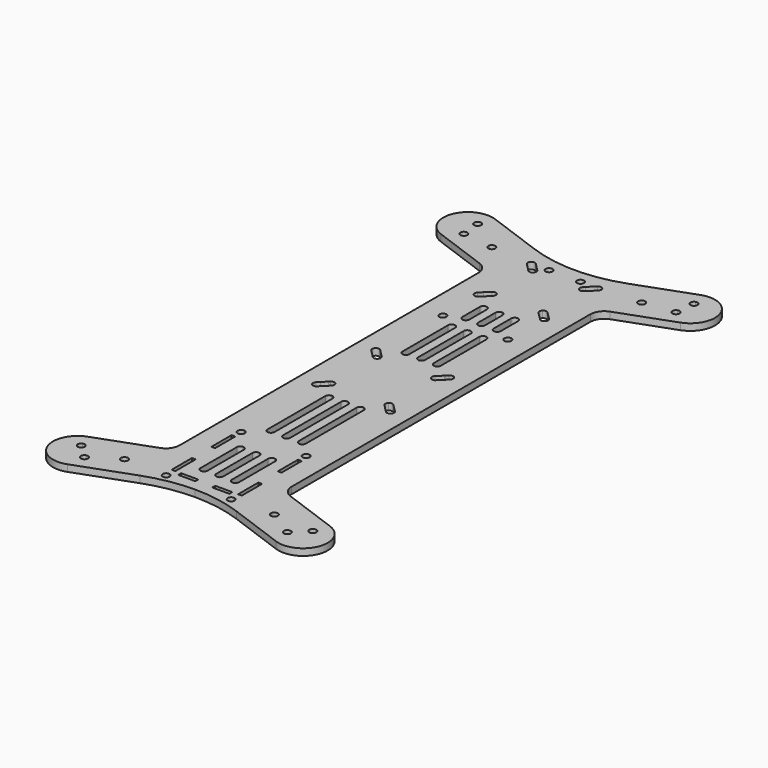
from build123d import *

# Parameters (mm, degrees)
F0_W     = 3.775
F0_H     = 1
F0_W_2   = 0.5
F0_H_2   = 10.85
F0_W_3   = 3.85
F0_H_3   = 25.4769915305
F0_H_4   = 9.7843557596
F0_H_5   = 20.2333889902
F1_DEPTH = 3


# Not quite as in the source:
# - a feature names something its author has since deleted; it is built from what else it names


with BuildPart() as f1:
    # F0 (on Top) → F1 (new body)
    with BuildSketch(Plane.XY):
        with Locations((6.6657602992, -80.0343685785)):
            Rectangle(F0_W, F0_H)
        with BuildLine():
            ThreePointArc((58.190047871, 117.9808986768), (64.7644140361, 132.0798244914), (50.6654338992, 138.6540741594))
            Line((50.6654338992, 138.6540741594), (52.5342574987, 133.5195235187))
            ThreePointArc((52.5342574987, 133.5195235187), (53.9763221117, 133.3296721108), (54.6479392245, 132.039507641))
            ThreePointArc((54.6479392245, 132.039507641), (54.3631036942, 131.1361247537), (53.6116209502, 130.5594917633))
            Line((53.6116209502, 130.5594917633), (54.7696756191, 127.37776271))
            Line((54.7696756191, 127.37776271), (58.190047871, 117.9808986768))
        make_face()
        with BuildLine():
            Line((36.7554780085, 120.8211309856), (29.7782602992, 118.2816314214))
            Line((29.778260321, 118.2816314276), (33.1987034785, 108.8847932036))
            Line((33.1987034785, 108.8847932036), (33.8827906821, 109.1337805834))
            Line((33.8827906821, 109.1337805834), (58.190047871, 117.9808986768))
            Line((58.190047871, 117.9808986768), (54.7696756191, 127.37776271))
            Line((54.7696756191, 127.37776271), (51.1158606394, 126.0478828159))
            Line((51.1158606394, 126.0478828159), (39.715509764, 121.8984944371))
            ThreePointArc((39.715509764, 121.8984944371), (39.7865660973, 121.6333085911), (39.8104938863, 121.3598127113))
            ThreePointArc((39.8104938863, 121.3598127113), (38.5089897661, 119.8087405003), (36.7554780085, 120.8211309856))
        make_face()
        with BuildLine():
            ThreePointArc((53.7365490928, 123.1748774023), (51.2581662055, 121.8847129326), (51.6228673671, 124.6548932801))
            ThreePointArc((51.6228673671, 124.6548932801), (53.06493198, 124.4650418721), (53.7365490928, 123.1748774023))
        make_face(mode=Mode.SUBTRACT)
        Polygon((33.1987034785, 108.8847932036), (29.778260321, 118.2816314276), (29.7782602992, 107.6398536984), align=None)
        with BuildLine():
            Line((14.9782756182, 115.4816467686), (9.7782603038, 110.2816314563))
            Line((9.7782603038, 110.2816314563), (9.7782603038, 100.281631451))
            Line((9.7782603038, 100.281631451), (14.9782756245, 95.0816161323))
            ThreePointArc((14.9782756245, 95.0816161323), (16.0919688055, 95.5429229525), (17.2056619867, 95.0816161328))
            Line((17.2056619867, 95.0816161328), (19.2782602992, 93.0090178203))
            Line((19.2782602992, 93.0090178203), (19.2782602992, 117.554245087))
            Line((19.2782602992, 117.554245087), (17.2056619804, 115.4816467682))
            ThreePointArc((17.2056619804, 115.4816467682), (16.0919687992, 115.0203399485), (14.9782756182, 115.4816467686))
        make_face()
        with BuildLine():
            Line((11.7782603087, 118.2816314214), (4.7782602992, 118.2816314214))
            Line((4.7782602992, 118.2816314214), (4.7782602992, 110.2816314563))
            Line((4.7782602992, 110.2816314563), (9.7782603038, 110.2816314563))
            Line((9.7782603038, 110.2816314563), (14.9782756182, 115.4816467686))
            ThreePointArc((14.9782756182, 115.4816467686), (14.5169687985, 116.5953399498), (14.9782756187, 117.7090331308))
            Line((14.9782756187, 117.7090331308), (15.5508739097, 118.2816314214))
            Line((15.5508739097, 118.2816314214), (11.7782603087, 118.2816314214))
        make_face()
        Polygon((9.7782603038, 110.2816314563), (4.7782602992, 110.2816314563), (4.7782602992, 105.2816314536), align=None)
        Polygon((9.7782603038, 110.2816314563), (4.7782602992, 105.2816314536), (9.7782603038, 100.281631451), align=None)
        Polygon((9.7782603038, 100.281631451), (4.7782602992, 105.2816314536), (4.7782602992, 100.281631451), align=None)
        with BuildLine():
            Line((9.7782603038, 100.281631451), (4.7782602992, 100.281631451))
            Line((4.7782602992, 100.281631451), (4.7782602992, 85.1705366492))
            ThreePointArc((4.7782602992, 85.1705366492), (5.8919534795, 84.7092298296), (6.3532602992, 83.5955366492))
            Line((6.3532602992, 83.5955366492), (10.2032602992, 83.5955366492))
            ThreePointArc((10.2032602992, 83.5955366492), (11.7782602992, 85.1705366492), (13.3532602992, 83.5955366492))
            Line((13.3532602992, 83.5955366492), (19.2782602992, 83.5955366492))
            Line((19.2782602992, 83.5955366492), (19.2782602992, 88.896597805))
            ThreePointArc((19.2782602992, 88.896597805), (18.866196709, 89.053607639), (18.5138095323, 89.3186958657))
            Line((18.5138095323, 89.3186958657), (14.978275625, 92.8542297702))
            ThreePointArc((14.978275625, 92.8542297702), (14.5169688048, 93.9679229512), (14.9782756245, 95.0816161323))
            Line((14.9782756245, 95.0816161323), (9.7782603038, 100.281631451))
        make_face()
        with BuildLine():
            Line((16.6290332129, 32.9517906959), (19.0508739384, 35.3736314215))
            Line((19.0508739384, 35.3736314215), (11.7782602992, 35.3736314215))
            Line((11.7782602992, 35.3736314215), (11.7782602992, 25.8736314215))
            Line((11.7782602992, 25.8736314215), (16.6290332129, 30.7244043352))
            ThreePointArc((16.6290332129, 30.7244043352), (16.1677263933, 31.8380975156), (16.6290332129, 32.9517906959))
        make_face()
        with BuildLine():
            Line((16.6290332129, 7.0228585078), (11.7782602992, 11.8736314215))
            Line((11.7782602992, 11.8736314215), (11.7782602992, 2.3736314215))
            Line((11.7782602992, 2.3736314215), (19.0508739384, 2.3736314215))
            Line((19.0508739384, 2.3736314215), (16.6290332129, 4.795472147))
            ThreePointArc((16.6290332129, 4.795472147), (16.1677263933, 5.9091653274), (16.6290332129, 7.0228585078))
        make_face()
        with BuildLine():
            Line((29.7782602992, -63.3962838112), (29.7782602992, 18.8736314215))
            Line((29.7782602992, 18.8736314215), (21.2782602992, 18.8736314215))
            Line((21.2782602992, 18.8736314215), (21.2782602992, 4.6010177822))
            Line((21.2782602992, 4.6010177822), (22.3919534795, 3.4873246019))
            ThreePointArc((22.3919534795, 3.4873246019), (22.7333705629, 2.9763578275), (22.8532602992, 2.3736314215))
            ThreePointArc((22.8532602992, 2.3736314215), (21.8809867051, 0.9185211578), (20.1645671188, 1.2599382411))
            Line((20.1645671188, 1.2599382411), (19.2782602992, 2.1462450608))
            Line((19.2782602992, 2.1462450608), (19.2782602992, -40.6093685785))
            ThreePointArc((19.2782602992, -40.6093685785), (20.3919534795, -41.0706753981), (20.8532602992, -42.1843685785))
            ThreePointArc((20.8532602992, -42.1843685785), (20.3919534795, -43.2980617588), (19.2782602992, -43.7593685785))
            Line((19.2782602992, -43.7593685785), (19.2782602992, -46.0843685785))
            Line((19.2782602992, -46.0843685785), (20.4282602992, -46.0843685785))
            Line((20.4282602992, -46.0843685785), (20.4282602992, -57.3843685785))
            Line((20.4282602992, -57.3843685785), (19.2782602992, -57.3843685785))
            Line((19.2782602992, -57.3843685785), (19.2782602992, -68.2343685785))
            Line((19.2782602992, -68.2343685785), (20.4282602992, -68.2343685785))
            Line((20.4282602992, -68.2343685785), (20.4282602992, -79.5343685785))
            Line((20.4282602992, -79.5343685785), (19.2782602992, -79.5343685785))
            Line((19.2782602992, -79.5343685785), (19.2782602992, -80.5343685785))
            Line((19.2782602992, -80.5343685785), (29.7782602992, -80.5343685785))
            Line((29.7782602992, -80.5343685785), (29.7782602992, -67.7642353088))
            Line((29.7782602992, -67.7642353088), (29.7782602992, -63.3962838112))
        make_face()
        with BuildLine():
            Line((19.0508739384, 2.3736314215), (11.7782602992, 2.3736314215))
            Line((11.7782602992, 2.3736314215), (11.7782602992, -1.0513685785))
            ThreePointArc((11.7782602992, -1.0513685785), (12.8919534795, -1.5126753981), (13.3532602992, -2.6263685785))
            Line((13.3532602992, -2.6263685785), (13.3532602992, -34.9310487509))
            ThreePointArc((13.3532602992, -34.9310487509), (12.8919534795, -36.0447419312), (11.7782602992, -36.5060487509))
            ThreePointArc((11.7782602992, -36.5060487509), (10.6645671188, -36.0447419312), (10.2032602992, -34.9310487509))
            Line((10.2032602992, -34.9310487509), (6.3532602992, -34.9310487509))
            ThreePointArc((6.3532602992, -34.9310487509), (5.8919534795, -36.0447419312), (4.7782602992, -36.5060487509))
            Line((4.7782602992, -36.5060487509), (4.7782602992, -46.0843685785))
            Line((4.7782602992, -46.0843685785), (18.7782602992, -46.0843685785))
            Line((18.7782602992, -46.0843685785), (19.2782602992, -46.0843685785))
            Line((19.2782602992, -46.0843685785), (19.2782602992, -43.7593685785))
            ThreePointArc((19.2782602992, -43.7593685785), (17.7032602992, -42.1843685785), (19.2782602992, -40.6093685785))
            Line((19.2782602992, -40.6093685785), (19.2782602992, 2.1462450608))
            Line((19.2782602992, 2.1462450608), (19.0508739384, 2.3736314215))
        make_face()
        with BuildLine():
            Line((-9.4943533401, 2.3736314215), (-9.7217397008, 2.1462450608))
            Line((-9.7217397008, 2.1462450608), (-9.7217397008, -40.6093685785))
            ThreePointArc((-9.7217397008, -40.6093685785), (-8.6080465205, -41.0706753981), (-8.1467397008, -42.1843685785))
            ThreePointArc((-8.1467397008, -42.1843685785), (-8.6080465205, -43.2980617588), (-9.7217397008, -43.7593685785))
            Line((-9.7217397008, -43.7593685785), (-9.7217397008, -46.0843685785))
            Line((-9.7217397008, -46.0843685785), (-9.2217397008, -46.0843685785))
            Line((-9.2217397008, -46.0843685785), (4.7782602992, -46.0843685785))
            Line((4.7782602992, -46.0843685785), (4.7782602992, -36.5060487509))
            ThreePointArc((4.7782602992, -36.5060487509), (3.6645671188, -36.0447419312), (3.2032602992, -34.9310487509))
            Line((3.2032602992, -34.9310487509), (-0.6467397008, -34.9310487509))
            ThreePointArc((-0.6467397008, -34.9310487509), (-1.1080465205, -36.0447419312), (-2.2217397008, -36.5060487509))
            ThreePointArc((-2.2217397008, -36.5060487509), (-3.3354328812, -36.0447419312), (-3.7967397008, -34.9310487509))
            Line((-3.7967397008, -34.9310487509), (-3.7967397008, -2.6263685785))
            ThreePointArc((-3.7967397008, -2.6263685785), (-3.3354328812, -1.5126753981), (-2.2217397008, -1.0513685785))
            Line((-2.2217397008, -1.0513685785), (-2.2217397008, 2.3736314215))
            Line((-2.2217397008, 2.3736314215), (-9.4943533401, 2.3736314215))
        make_face()
        Polygon((4.7782602992, 100.281631451), (4.7782602992, 105.2816314536), (-0.2217397055, 100.281631451), align=None)
        with BuildLine():
            Line((26.358348936, -89.9314003632), (29.7782602992, -80.5343685785))
            Line((29.7782602992, -80.5343685785), (19.2782602992, -80.5343685785))
            Line((19.2782602992, -80.5343685785), (16.2032602992, -80.5343685785))
            Line((16.2032602992, -80.5343685785), (16.2032602992, -81.1843685785))
            Line((16.2032602992, -81.1843685785), (8.5532602992, -81.1843685785))
            Line((8.5532602992, -81.1843685785), (8.5532602992, -80.5343685785))
            Line((8.5532602992, -80.5343685785), (4.7782602992, -80.5343685785))
            Line((4.7782602992, -80.5343685785), (1.0032602992, -80.5343685785))
            Line((1.0032602992, -80.5343685785), (1.0032602992, -81.1843685785))
            Line((1.0032602992, -81.1843685785), (-6.6467397008, -81.1843685785))
            Line((-6.6467397008, -81.1843685785), (-6.6467397008, -80.5343685785))
            Line((-6.6467397008, -80.5343685785), (-9.7217397008, -80.5343685785))
            Line((-9.7217397008, -80.5343685785), (-20.2217397008, -80.5343685785))
            Line((-20.2217397008, -80.5343685785), (-16.8018283377, -89.9314003632))
            ThreePointArc((-16.8018283377, -89.9314003632), (-6.1782378405, -87.0848178692), (4.7782603087, -86.1262484905))
            ThreePointArc((4.7782602897, -86.1262484905), (15.7347584389, -87.0848178692), (26.358348936, -89.9314003632))
        make_face()
        with BuildLine():
            ThreePointArc((-8.1467397008, -84.0343685785), (-10.8354328812, -85.1480617588), (-9.7217397008, -82.4593685785))
            ThreePointArc((-9.7217397008, -82.4593685785), (-8.6080465205, -82.9206753981), (-8.1467397008, -84.0343685785))
        make_face(mode=Mode.SUBTRACT)
        with BuildLine():
            ThreePointArc((20.8532602992, -84.0343685785), (18.1645671188, -85.1480617588), (19.2782602992, -82.4593685785))
            ThreePointArc((19.2782602992, -82.4593685785), (20.3919534795, -82.9206753981), (20.8532602992, -84.0343685785))
        make_face(mode=Mode.SUBTRACT)
        with BuildLine():
            ThreePointArc((33.8827920894, -69.258162706), (30.9064045362, -66.9743002098), (29.7782602992, -63.3962838112))
            Line((29.7782602992, -63.3962838112), (29.7782602992, -67.7642353088))
            Line((29.7782602992, -67.7642353088), (33.8827920894, -69.258162706))
        make_face()
        Polygon((33.8827920894, -69.258162706), (29.7782602992, -67.7642353088), (29.7782602992, -80.5343685785), align=None)
        with BuildLine():
            Line((36.7554780085, -83.0738681427), (29.7782602992, -80.5343685785))
            Line((29.7782602992, -80.5343685785), (26.358348936, -89.9314003632))
            Line((26.358348936, -89.9314003632), (51.3494741858, -99.027426075))
            Line((51.3494741858, -99.027426075), (54.7696756191, -89.6304998671))
            Line((54.7696756191, -89.6304998671), (51.1158606393, -88.3006199729))
            Line((51.1158606393, -88.3006199729), (39.715509764, -84.1512315941))
            ThreePointArc((39.715509764, -84.1512315941), (37.6968121605, -85.0925657461), (36.7554780085, -83.0738681427))
        make_face()
        with BuildLine():
            ThreePointArc((51.6451721859, -91.1736253865), (48.7800077162, -92.0770082738), (50.6088539116, -89.6936095088))
            ThreePointArc((50.6088539116, -89.6936095088), (51.3603366557, -90.2702424993), (51.6451721859, -91.1736253865))
        make_face(mode=Mode.SUBTRACT)
        with BuildLine():
            Line((58.873917339, -78.3541884177), (33.8827920894, -69.258162706))
            Line((33.8827920894, -69.258162706), (29.7782602992, -80.5343685785))
            Line((29.7782602992, -80.5343685785), (36.7554780085, -83.0738681427))
            ThreePointArc((36.7554780085, -83.0738681427), (38.5089897661, -82.0614776574), (39.8104938862, -83.6125498684))
            ThreePointArc((39.8104938862, -83.6125498684), (39.7865660972, -83.8860457482), (39.715509764, -84.1512315941))
            Line((39.715509764, -84.1512315941), (51.1158606393, -88.3006199729))
            Line((51.1158606393, -88.3006199729), (54.7696756191, -89.6304998671))
            Line((54.7696756191, -89.6304998671), (55.927730288, -86.4487708139))
            ThreePointArc((55.927730288, -86.4487708139), (54.9863961359, -84.4300732104), (57.0050937394, -83.4887390584))
            Line((57.0050937394, -83.4887390584), (58.873917339, -78.3541884177))
        make_face()
        with BuildLine():
            ThreePointArc((51.3494741858, -99.027426075), (65.4483145911, -92.4530288229), (58.873917339, -78.3541884177))
            Line((58.873917339, -78.3541884177), (57.0050937394, -83.4887390584))
            ThreePointArc((57.0050937394, -83.4887390584), (57.7565764834, -84.0653720489), (58.0414120137, -84.9687549362))
            ThreePointArc((58.0414120137, -84.9687549362), (57.3697949009, -86.2589194059), (55.927730288, -86.4487708139))
            Line((55.927730288, -86.4487708139), (54.7696756191, -89.6304998671))
            Line((54.7696756191, -89.6304998671), (51.3494741858, -99.027426075))
        make_face()
        Polygon((16.2032602992, -80.5343685785), (19.2782602992, -80.5343685785), (19.2782602992, -79.5343685785), (18.7782602992, -79.5343685785), (16.2032602992, -79.5343685785), align=None)
        with Locations((19.0282602992, -62.8093685785)):
            Rectangle(F0_W_2, F0_H_2)
        with BuildLine():
            Line((-23.6421828801, 108.8847932036), (-20.2217397227, 118.2816314276))
            Line((-20.2217397008, 118.2816314214), (-27.1989574102, 120.8211309856))
            ThreePointArc((-27.1989574102, 120.8211309856), (-29.2176550137, 119.8797968336), (-30.1589891657, 121.8984944371))
            Line((-30.1589891657, 121.8984944371), (-41.559340041, 126.0478828159))
            Line((-41.559340041, 126.0478828159), (-45.2131550207, 127.37776271))
            Line((-45.2131550207, 127.37776271), (-48.6335272726, 117.9808986768))
            Line((-48.6335272726, 117.9808986768), (-24.3262700838, 109.1337805834))
            Line((-24.3262700838, 109.1337805834), (-23.6421828801, 108.8847932036))
        make_face()
        with BuildLine():
            ThreePointArc((-41.0300284945, 123.1748774023), (-43.8951929642, 122.2714945151), (-42.0663467687, 124.6548932801))
            ThreePointArc((-42.0663467687, 124.6548932801), (-41.3148640247, 124.0782602896), (-41.0300284945, 123.1748774023))
        make_face(mode=Mode.SUBTRACT)
        with BuildLine():
            Line((-27.1989574102, 120.8211309856), (-20.2217397008, 118.2816314214))
            Line((-20.2217397008, 118.2816314214), (-16.117846067, 129.5580695577))
            Line((-16.117846067, 129.5580695577), (-41.1089133008, 138.6540741594))
            Line((-41.1089133008, 138.6540741594), (-42.9777369004, 133.5195235187))
            ThreePointArc((-42.9777369004, 133.5195235187), (-42.2262541564, 132.9428905283), (-41.9414186261, 132.039507641))
            ThreePointArc((-41.9414186261, 132.039507641), (-42.6130357389, 130.7493431712), (-44.0551003519, 130.5594917633))
            Line((-44.0551003519, 130.5594917633), (-45.2131550207, 127.37776271))
            Line((-45.2131550207, 127.37776271), (-41.559340041, 126.0478828159))
            Line((-41.559340041, 126.0478828159), (-30.1589891657, 121.8984944371))
            ThreePointArc((-30.1589891657, 121.8984944371), (-28.4054774081, 122.9108849223), (-27.1039732879, 121.3598127113))
            ThreePointArc((-27.1039732879, 121.3598127113), (-27.1279010769, 121.0863168315), (-27.1989574102, 120.8211309856))
        make_face()
        with BuildLine():
            Line((-42.9777369004, 133.5195235187), (-41.1089133008, 138.6540741594))
            ThreePointArc((-41.1089133008, 138.6540741594), (-55.2078934377, 132.0798244914), (-48.6335272726, 117.9808986768))
            Line((-48.6335272726, 117.9808986768), (-45.2131550207, 127.37776271))
            Line((-45.2131550207, 127.37776271), (-44.0551003519, 130.5594917633))
            ThreePointArc((-44.0551003519, 130.5594917633), (-44.9964345039, 132.5781893667), (-42.9777369004, 133.5195235187))
        make_face()
        with BuildLine():
            Line((-9.7217397008, 93.0090178203), (-9.7217397008, 117.554245087))
            Line((-9.7217397008, 117.554245087), (-10.4491260352, 118.2816314214))
            Line((-10.4491260352, 118.2816314214), (-20.2217397008, 118.2816314214))
            Line((-20.2217397008, 118.2816314214), (-20.2217397008, 107.6398536984))
            Line((-20.2217397008, 107.6398536984), (-20.2217397008, 103.2719036984))
            Line((-20.2217397008, 103.2719036984), (-20.2217397008, 18.8736314215))
            Line((-20.2217397008, 18.8736314215), (-11.7217397008, 18.8736314215))
            Line((-11.7217397008, 18.8736314215), (-11.7217397008, 33.1462450607))
            Line((-11.7217397008, 33.1462450607), (-12.8354328812, 34.2599382411))
            ThreePointArc((-12.8354328812, 34.2599382411), (-12.8354328812, 36.4873246018), (-10.6080465204, 36.4873246018))
            Line((-10.6080465204, 36.4873246018), (-9.7217397008, 35.6010177822))
            Line((-9.7217397008, 35.6010177822), (-9.7217397008, 40.3736314215))
            Line((-9.7217397008, 40.3736314215), (-9.7217397008, 68.7986314215))
            ThreePointArc((-9.7217397008, 68.7986314215), (-11.2967397008, 70.3736314215), (-9.7217397008, 71.9486314215))
            Line((-9.7217397008, 71.9486314215), (-9.7217397008, 83.5955366492))
            Line((-9.7217397008, 83.5955366492), (-9.7217397008, 88.896597805))
            ThreePointArc((-9.7217397008, 88.896597805), (-11.4497635214, 89.6710830428), (-11.1846752943, 91.5460822269))
            Line((-11.1846752943, 91.5460822269), (-9.7217397008, 93.0090178203))
        make_face()
        with BuildLine():
            Line((-0.2217397055, 100.281631451), (-0.2217397055, 110.2816314563))
            Line((-0.2217397055, 110.2816314563), (-5.4217550199, 115.4816467686))
            ThreePointArc((-5.4217550199, 115.4816467686), (-6.5354482008, 115.0203399485), (-7.649141382, 115.4816467682))
            Line((-7.649141382, 115.4816467682), (-9.7217397008, 117.554245087))
            Line((-9.7217397008, 117.554245087), (-9.7217397008, 93.0090178203))
            Line((-9.7217397008, 93.0090178203), (-7.6491413883, 95.0816161328))
            ThreePointArc((-7.6491413883, 95.0816161328), (-6.5354482072, 95.5429229525), (-5.4217550262, 95.0816161323))
            Line((-5.4217550262, 95.0816161323), (-0.2217397055, 100.281631451))
        make_face()
        with BuildLine():
            Line((4.7782602992, 110.2816314563), (4.7782602992, 118.2816314214))
            Line((4.7782602992, 118.2816314214), (-2.2217397103, 118.2816314214))
            Line((-2.2217397103, 118.2816314214), (-5.9943533114, 118.2816314214))
            Line((-5.9943533114, 118.2816314214), (-5.4217550203, 117.7090331308))
            ThreePointArc((-5.4217550203, 117.7090331308), (-5.0803379366, 117.198066356), (-4.9604482002, 116.5953399495))
            ThreePointArc((-4.9604482002, 116.5953399495), (-5.0803379365, 115.9926135432), (-5.4217550199, 115.4816467686))
            Line((-5.4217550199, 115.4816467686), (-0.2217397055, 110.2816314563))
            Line((-0.2217397055, 110.2816314563), (4.7782602992, 110.2816314563))
        make_face()
        with BuildLine():
            Line((20.0056466336, 118.2816314214), (19.2782602992, 117.554245087))
            Line((19.2782602992, 117.554245087), (19.2782602992, 93.0090178203))
            Line((19.2782602992, 93.0090178203), (20.7411958926, 91.5460822269))
            ThreePointArc((20.7411958926, 91.5460822269), (21.0826129761, 91.0351154524), (21.2025027125, 90.4323890463))
            ThreePointArc((21.2025027125, 90.4323890463), (20.6099914399, 89.2013972102), (19.2782602992, 88.896597805))
            Line((19.2782602992, 88.896597805), (19.2782602992, 83.5955366492))
            Line((19.2782602992, 83.5955366492), (19.2782602992, 71.9486314215))
            ThreePointArc((19.2782602992, 71.9486314215), (20.3919534795, 71.4873246018), (20.8532602992, 70.3736314215))
            ThreePointArc((20.8532602992, 70.3736314215), (20.3919534795, 69.2599382411), (19.2782602992, 68.7986314215))
            Line((19.2782602992, 68.7986314215), (19.2782602992, 40.3736314215))
            Line((19.2782602992, 40.3736314215), (19.2782602992, 35.6010177822))
            Line((19.2782602992, 35.6010177822), (20.1645671188, 36.4873246018))
            ThreePointArc((20.1645671188, 36.4873246018), (21.8809867051, 36.8287416852), (22.8532602992, 35.3736314215))
            ThreePointArc((22.8532602992, 35.3736314215), (22.7333705629, 34.7709050155), (22.3919534795, 34.2599382411))
            Line((22.3919534795, 34.2599382411), (21.2782602992, 33.1462450607))
            Line((21.2782602992, 33.1462450607), (21.2782602992, 18.8736314215))
            Line((21.2782602992, 18.8736314215), (29.7782602992, 18.8736314215))
            Line((29.7782602992, 18.8736314215), (29.7782602992, 103.2719036984))
            Line((29.7782602992, 103.2719036984), (29.7782602992, 107.6398536984))
            Line((29.7782602992, 107.6398536984), (29.7782602992, 118.2816314214))
            Line((29.7782602992, 118.2816314214), (20.0056466336, 118.2816314214))
        make_face()
        with BuildLine():
            Line((4.7782602992, 85.1705366492), (4.7782602992, 100.281631451))
            Line((4.7782602992, 100.281631451), (-0.2217397055, 100.281631451))
            Line((-0.2217397055, 100.281631451), (-5.4217550262, 95.0816161323))
            ThreePointArc((-5.4217550262, 95.0816161323), (-5.0803379428, 94.5706493577), (-4.9604482065, 93.9679229515))
            ThreePointArc((-4.9604482065, 93.9679229515), (-5.0803379429, 93.365196545), (-5.4217550266, 92.8542297702))
            Line((-5.4217550266, 92.8542297702), (-8.957288934, 89.3186958657))
            ThreePointArc((-8.957288934, 89.3186958657), (-9.3096761107, 89.053607639), (-9.7217397008, 88.896597805))
            Line((-9.7217397008, 88.896597805), (-9.7217397008, 83.5955366492))
            Line((-9.7217397008, 83.5955366492), (-3.7967397008, 83.5955366492))
            ThreePointArc((-3.7967397008, 83.5955366492), (-2.2217397008, 85.1705366492), (-0.6467397008, 83.5955366492))
            Line((-0.6467397008, 83.5955366492), (3.2032602992, 83.5955366492))
            ThreePointArc((3.2032602992, 83.5955366492), (3.6645671188, 84.7092298296), (4.7782602992, 85.1705366492))
        make_face()
        Polygon((4.7782602992, 105.2816314536), (4.7782602992, 110.2816314563), (-0.2217397055, 110.2816314563), align=None)
        Polygon((-0.2217397055, 100.281631451), (4.7782602992, 105.2816314536), (-0.2217397055, 110.2816314563), align=None)
        with BuildLine():
            Line((-2.2217397008, 35.3736314215), (-9.4943533401, 35.3736314215))
            Line((-9.4943533401, 35.3736314215), (-7.0725126145, 32.9517906959))
            ThreePointArc((-7.0725126145, 32.9517906959), (-6.7310955312, 32.4408239215), (-6.6112057949, 31.8380975156))
            ThreePointArc((-6.6112057949, 31.8380975156), (-6.7310955312, 31.2353711096), (-7.0725126145, 30.7244043352))
            Line((-7.0725126145, 30.7244043352), (-2.2217397008, 25.8736314215))
            Line((-2.2217397008, 25.8736314215), (-2.2217397008, 35.3736314215))
        make_face()
        with BuildLine():
            Line((-9.7217397008, 31.1462450607), (-9.7217397008, 18.8736314215))
            Line((-9.7217397008, 18.8736314215), (-2.2217397008, 18.8736314215))
            Line((-2.2217397008, 18.8736314215), (-2.2217397008, 25.8736314215))
            Line((-2.2217397008, 25.8736314215), (-7.0725126145, 30.7244043352))
            ThreePointArc((-7.0725126145, 30.7244043352), (-8.1862057949, 30.2630975156), (-9.2998989753, 30.7244043352))
            Line((-9.2998989753, 30.7244043352), (-9.7217397008, 31.1462450607))
        make_face()
        with BuildLine():
            Line((-2.2217397008, 18.8736314215), (-9.7217397008, 18.8736314215))
            Line((-9.7217397008, 18.8736314215), (-9.7217397008, 6.6010177822))
            Line((-9.7217397008, 6.6010177822), (-9.2998989753, 7.0228585078))
            ThreePointArc((-9.2998989753, 7.0228585078), (-8.1862057949, 7.4841653274), (-7.0725126145, 7.0228585078))
            Line((-7.0725126145, 7.0228585078), (-2.2217397008, 11.8736314215))
            Line((-2.2217397008, 11.8736314215), (-2.2217397008, 18.8736314215))
        make_face()
        with BuildLine():
            Line((-2.2217397008, 2.3736314215), (-2.2217397008, 11.8736314215))
            Line((-2.2217397008, 11.8736314215), (-7.0725126145, 7.0228585078))
            ThreePointArc((-7.0725126145, 7.0228585078), (-6.7310955312, 6.5118917334), (-6.6112057949, 5.9091653274))
            ThreePointArc((-6.6112057949, 5.9091653274), (-6.7310955312, 5.3064389214), (-7.0725126145, 4.795472147))
            Line((-7.0725126145, 4.795472147), (-9.4943533401, 2.3736314215))
            Line((-9.4943533401, 2.3736314215), (-2.2217397008, 2.3736314215))
        make_face()
        with BuildLine():
            Line((11.7782602992, 18.8736314215), (19.2782602992, 18.8736314215))
            Line((19.2782602992, 18.8736314215), (19.2782602992, 31.1462450607))
            Line((19.2782602992, 31.1462450607), (18.8564195736, 30.7244043352))
            ThreePointArc((18.8564195736, 30.7244043352), (17.7427263933, 30.2630975156), (16.6290332129, 30.7244043352))
            Line((16.6290332129, 30.7244043352), (11.7782602992, 25.8736314215))
            Line((11.7782602992, 25.8736314215), (11.7782602992, 18.8736314215))
        make_face()
        with BuildLine():
            Line((19.2782602992, 6.6010177822), (19.2782602992, 18.8736314215))
            Line((19.2782602992, 18.8736314215), (11.7782602992, 18.8736314215))
            Line((11.7782602992, 18.8736314215), (11.7782602992, 11.8736314215))
            Line((11.7782602992, 11.8736314215), (16.6290332129, 7.0228585078))
            ThreePointArc((16.6290332129, 7.0228585078), (17.7427263933, 7.4841653274), (18.8564195736, 7.0228585078))
            Line((18.8564195736, 7.0228585078), (19.2782602992, 6.6010177822))
        make_face()
        Polygon((19.2782602992, 18.8736314215), (21.2782602992, 18.8736314215), (21.2782602992, 33.1462450607), (19.2782602992, 31.1462450607), align=None)
        Polygon((21.2782602992, 4.6010177822), (21.2782602992, 18.8736314215), (19.2782602992, 18.8736314215), (19.2782602992, 6.6010177822), align=None)
        Polygon((-9.7217397008, 18.8736314215), (-11.7217397008, 18.8736314215), (-11.7217397008, 4.6010177822), (-9.7217397008, 6.6010177822), align=None)
        Polygon((-11.7217397008, 33.1462450607), (-11.7217397008, 18.8736314215), (-9.7217397008, 18.8736314215), (-9.7217397008, 31.1462450607), align=None)
        with BuildLine():
            Line((-20.2217397008, -80.5343685785), (-24.3262714911, -69.258162706))
            Line((-24.3262714911, -69.258162706), (-49.3173967406, -78.3541884177))
            Line((-49.3173967406, -78.3541884177), (-47.4485731411, -83.4887390584))
            ThreePointArc((-47.4485731411, -83.4887390584), (-46.0065085281, -83.6785904664), (-45.3348914153, -84.9687549362))
            ThreePointArc((-45.3348914153, -84.9687549362), (-45.6197269456, -85.8721378234), (-46.3712096896, -86.4487708139))
            Line((-46.3712096896, -86.4487708139), (-45.2131550207, -89.6304998671))
            Line((-45.2131550207, -89.6304998671), (-41.559340041, -88.3006199729))
            Line((-41.559340041, -88.3006199729), (-30.1589891656, -84.1512315941))
            ThreePointArc((-30.1589891656, -84.1512315941), (-29.2176550136, -82.1325339907), (-27.1989574102, -83.0738681427))
            Line((-27.1989574102, -83.0738681427), (-20.2217397008, -80.5343685785))
        make_face()
        with BuildLine():
            Line((-16.8018283377, -89.9314003632), (-20.2217397008, -80.5343685785))
            Line((-20.2217397008, -80.5343685785), (-27.1989574102, -83.0738681427))
            ThreePointArc((-27.1989574102, -83.0738681427), (-27.1279010769, -83.3390539886), (-27.1039732879, -83.6125498684))
            ThreePointArc((-27.1039732879, -83.6125498684), (-28.4054774081, -85.1636220794), (-30.1589891656, -84.1512315941))
            Line((-30.1589891656, -84.1512315941), (-41.559340041, -88.3006199729))
            Line((-41.559340041, -88.3006199729), (-45.2131550207, -89.6304998671))
            Line((-45.2131550207, -89.6304998671), (-41.7929535875, -99.027426075))
            Line((-41.7929535875, -99.027426075), (-16.8018283377, -89.9314003632))
        make_face()
        with BuildLine():
            ThreePointArc((-38.9386515876, -91.1736253865), (-41.4170344748, -92.4637898563), (-41.0523333133, -89.6936095088))
            ThreePointArc((-41.0523333133, -89.6936095088), (-39.6102687003, -89.8834609168), (-38.9386515876, -91.1736253865))
        make_face(mode=Mode.SUBTRACT)
        with BuildLine():
            Line((-47.4485731411, -83.4887390584), (-49.3173967406, -78.3541884177))
            ThreePointArc((-49.3173967406, -78.3541884177), (-55.8917939927, -92.4530288229), (-41.7929535875, -99.027426075))
            Line((-41.7929535875, -99.027426075), (-45.2131550207, -89.6304998671))
            Line((-45.2131550207, -89.6304998671), (-46.3712096896, -86.4487708139))
            ThreePointArc((-46.3712096896, -86.4487708139), (-48.3899072931, -85.5074366619), (-47.4485731411, -83.4887390584))
        make_face()
        Polygon((-20.2217397008, -67.7642353088), (-24.3262714911, -69.258162706), (-20.2217397008, -80.5343685785), align=None)
        with BuildLine():
            Line((-20.2217397008, -67.7642353088), (-20.2217397008, -63.3962838112))
            ThreePointArc((-20.2217397008, -63.3962838112), (-21.3498839379, -66.9743002098), (-24.3262714911, -69.258162706))
            Line((-24.3262714911, -69.258162706), (-20.2217397008, -67.7642353088))
        make_face()
        with Locations((2.8907602992, -80.0343685785)):
            Rectangle(F0_W, F0_H)
        Polygon((-9.7217397008, -79.5343685785), (-9.7217397008, -80.5343685785), (-6.6467397008, -80.5343685785), (-6.6467397008, -79.5343685785), (-9.2217397008, -79.5343685785), align=None)
        with BuildLine():
            Line((-11.7217397008, 18.8736314215), (-20.2217397008, 18.8736314215))
            Line((-20.2217397008, 18.8736314215), (-20.2217397008, -63.3962838112))
            Line((-20.2217397008, -63.3962838112), (-20.2217397008, -67.7642353088))
            Line((-20.2217397008, -67.7642353088), (-20.2217397008, -80.5343685785))
            Line((-20.2217397008, -80.5343685785), (-9.7217397008, -80.5343685785))
            Line((-9.7217397008, -80.5343685785), (-9.7217397008, -79.5343685785))
            Line((-9.7217397008, -79.5343685785), (-10.8717397008, -79.5343685785))
            Line((-10.8717397008, -79.5343685785), (-10.8717397008, -68.2343685785))
            Line((-10.8717397008, -68.2343685785), (-9.7217397008, -68.2343685785))
            Line((-9.7217397008, -68.2343685785), (-9.7217397008, -57.3843685785))
            Line((-9.7217397008, -57.3843685785), (-10.8717397008, -57.3843685785))
            Line((-10.8717397008, -57.3843685785), (-10.8717397008, -46.0843685785))
            Line((-10.8717397008, -46.0843685785), (-9.7217397008, -46.0843685785))
            Line((-9.7217397008, -46.0843685785), (-9.7217397008, -43.7593685785))
            ThreePointArc((-9.7217397008, -43.7593685785), (-11.2967397008, -42.1843685785), (-9.7217397008, -40.6093685785))
            Line((-9.7217397008, -40.6093685785), (-9.7217397008, 2.1462450608))
            Line((-9.7217397008, 2.1462450608), (-10.6080465204, 1.2599382411))
            ThreePointArc((-10.6080465204, 1.2599382411), (-12.8354328812, 1.2599382411), (-12.8354328812, 3.4873246019))
            Line((-12.8354328812, 3.4873246019), (-11.7217397008, 4.6010177822))
            Line((-11.7217397008, 4.6010177822), (-11.7217397008, 18.8736314215))
        make_face()
        with Locations((-9.4717397008, -62.8093685785)):
            Rectangle(F0_W_2, F0_H_2)
        with BuildLine():
            Line((-2.2217397103, 118.2816314214), (4.7782602992, 118.2816314214))
            Line((4.7782602992, 118.2816314214), (11.7782603087, 118.2816314214))
            Line((11.7782603087, 118.2816314214), (15.5508739097, 118.2816314214))
            Line((15.5508739097, 118.2816314214), (18.5138095274, 121.2445670367))
            ThreePointArc((18.5138095274, 121.2445670367), (20.2302291137, 121.5859841197), (21.2025027076, 120.1308738561))
            ThreePointArc((21.2025027076, 120.1308738561), (21.0826129712, 119.52814745), (20.7411958877, 119.0171806755))
            Line((20.7411958877, 119.0171806755), (20.0056466336, 118.2816314214))
            Line((20.0056466336, 118.2816314214), (29.7782602992, 118.2816314214))
            Line((29.7782602992, 118.2816314214), (25.6740185792, 129.5579428708))
            ThreePointArc((25.6740185792, 129.5579428708), (4.7780750868, 125.8734569022), (-16.117846067, 129.5580695577))
            Line((-16.117846067, 129.5580695577), (-20.2217397008, 118.2816314214))
            Line((-20.2217397008, 118.2816314214), (-10.4491260352, 118.2816314214))
            Line((-10.4491260352, 118.2816314214), (-11.1846752894, 119.0171806755))
            ThreePointArc((-11.1846752894, 119.0171806755), (-11.1846752898, 121.2445670362), (-8.9572889291, 121.2445670367))
            Line((-8.9572889291, 121.2445670367), (-5.9943533114, 118.2816314214))
            Line((-5.9943533114, 118.2816314214), (-2.2217397103, 118.2816314214))
        make_face()
        with BuildLine():
            ThreePointArc((-0.6467397103, 120.2816314549), (-1.10804653, 119.1679382745), (-2.2217397103, 118.7066314549))
            ThreePointArc((-2.2217397103, 118.7066314549), (-3.3354328907, 121.3953246352), (-0.6467397103, 120.2816314549))
        make_face(mode=Mode.SUBTRACT)
        with BuildLine():
            ThreePointArc((13.3532603087, 120.2816314549), (12.891953489, 119.1679382745), (11.7782603087, 118.7066314549))
            ThreePointArc((11.7782603087, 118.7066314549), (10.6645671283, 121.3953246352), (13.3532603087, 120.2816314549))
        make_face(mode=Mode.SUBTRACT)
        with BuildLine():
            Line((25.6740185792, 129.5579428708), (29.7782602992, 118.2816314214))
            Line((29.7782602992, 118.2816314214), (36.7554780085, 120.8211309856))
            ThreePointArc((36.7554780085, 120.8211309856), (37.6968121605, 122.8398285891), (39.715509764, 121.8984944371))
            Line((39.715509764, 121.8984944371), (51.1158606394, 126.0478828159))
            Line((51.1158606394, 126.0478828159), (54.7696756191, 127.37776271))
            Line((54.7696756191, 127.37776271), (53.6116209502, 130.5594917633))
            ThreePointArc((53.6116209502, 130.5594917633), (51.5929233467, 131.5008259153), (52.5342574987, 133.5195235187))
            Line((52.5342574987, 133.5195235187), (50.6654338992, 138.6540741594))
            Line((50.6654338992, 138.6540741594), (25.6740185792, 129.5579428708))
        make_face()
        Polygon((-20.2217397008, 107.6398536984), (-20.2217397008, 118.2816314214), (-23.6421828801, 108.8847932036), align=None)
        with BuildLine():
            Line((-20.2217397008, 107.6398536984), (-23.6421828801, 108.8847932036))
            Line((-23.6421828801, 108.8847932036), (-24.3262700838, 109.1337805834))
            ThreePointArc((-24.3262700838, 109.1337805834), (-21.3498835511, 106.8499188702), (-20.2217397008, 103.2719036984))
            Line((-20.2217397008, 103.2719036984), (-20.2217397008, 107.6398536984))
        make_face()
        with BuildLine():
            Line((33.1987034785, 108.8847932036), (29.7782602992, 107.6398536984))
            Line((29.7782602992, 107.6398536984), (29.7782602992, 103.2719036984))
            ThreePointArc((29.7782602992, 103.2719036984), (30.9064041494, 106.8499188702), (33.8827906821, 109.1337805834))
            Line((33.8827906821, 109.1337805834), (33.1987034785, 108.8847932036))
        make_face()
        with BuildLine():
            Line((8.5532602992, -79.5343685785), (16.2032602992, -79.5343685785))
            Line((16.2032602992, -79.5343685785), (18.7782602992, -79.5343685785))
            Line((18.7782602992, -79.5343685785), (18.7782602992, -68.2343685785))
            Line((18.7782602992, -68.2343685785), (18.7782602992, -57.3843685785))
            Line((18.7782602992, -57.3843685785), (18.7782602992, -46.0843685785))
            Line((18.7782602992, -46.0843685785), (4.7782602992, -46.0843685785))
            Line((4.7782602992, -46.0843685785), (4.7782602992, -50.4953308284))
            ThreePointArc((4.7782602992, -50.4953308284), (5.8919534795, -50.9566376481), (6.3532602992, -52.0703308284))
            Line((6.3532602992, -52.0703308284), (10.2032602992, -52.0703308284))
            ThreePointArc((10.2032602992, -52.0703308284), (10.6645671188, -50.9566376481), (11.7782602992, -50.4953308284))
            ThreePointArc((11.7782602992, -50.4953308284), (12.8919534795, -50.9566376481), (13.3532602992, -52.0703308284))
            Line((13.3532602992, -52.0703308284), (13.3532602992, -72.3037198186))
            ThreePointArc((13.3532602992, -72.3037198186), (11.7782602992, -73.8787198186), (10.2032602992, -72.3037198186))
            Line((10.2032602992, -72.3037198186), (6.3532602992, -72.3037198186))
            ThreePointArc((6.3532602992, -72.3037198186), (5.8919534795, -73.417412999), (4.7782602992, -73.8787198186))
            Line((4.7782602992, -73.8787198186), (4.7782602992, -79.5343685785))
            Line((4.7782602992, -79.5343685785), (8.5532602992, -79.5343685785))
        make_face()
        with BuildLine():
            Line((-9.2217397008, -68.2343685785), (-9.2217397008, -79.5343685785))
            Line((-9.2217397008, -79.5343685785), (-6.6467397008, -79.5343685785))
            Line((-6.6467397008, -79.5343685785), (1.0032602992, -79.5343685785))
            Line((1.0032602992, -79.5343685785), (4.7782602992, -79.5343685785))
            Line((4.7782602992, -79.5343685785), (4.7782602992, -73.8787198186))
            ThreePointArc((4.7782602992, -73.8787198186), (3.6645671188, -73.417412999), (3.2032602992, -72.3037198186))
            Line((3.2032602992, -72.3037198186), (-0.6467397008, -72.3037198186))
            ThreePointArc((-0.6467397008, -72.3037198186), (-2.2217397008, -73.8787198186), (-3.7967397008, -72.3037198186))
            Line((-3.7967397008, -72.3037198186), (-3.7967397008, -52.0703308284))
            ThreePointArc((-3.7967397008, -52.0703308284), (-3.3354328812, -50.9566376481), (-2.2217397008, -50.4953308284))
            ThreePointArc((-2.2217397008, -50.4953308284), (-1.1080465205, -50.9566376481), (-0.6467397008, -52.0703308284))
            Line((-0.6467397008, -52.0703308284), (3.2032602992, -52.0703308284))
            ThreePointArc((3.2032602992, -52.0703308284), (3.6645671188, -50.9566376481), (4.7782602992, -50.4953308284))
            Line((4.7782602992, -50.4953308284), (4.7782602992, -46.0843685785))
            Line((4.7782602992, -46.0843685785), (-9.2217397008, -46.0843685785))
            Line((-9.2217397008, -46.0843685785), (-9.2217397008, -57.3843685785))
            Line((-9.2217397008, -57.3843685785), (-9.2217397008, -68.2343685785))
        make_face()
        with BuildLine():
            Line((10.2032602992, 73.8111808896), (6.3532602992, 73.8111808896))
            ThreePointArc((6.3532602992, 73.8111808896), (4.7782602992, 72.2361808896), (3.2032602992, 73.8111808896))
            Line((3.2032602992, 73.8111808896), (-0.6467397008, 73.8111808896))
            ThreePointArc((-0.6467397008, 73.8111808896), (-2.2217397008, 72.2361808896), (-3.7967397008, 73.8111808896))
            Line((-3.7967397008, 73.8111808896), (-3.7967397008, 83.5955366492))
            Line((-3.7967397008, 83.5955366492), (-9.7217397008, 83.5955366492))
            Line((-9.7217397008, 83.5955366492), (-9.7217397008, 71.9486314215))
            ThreePointArc((-9.7217397008, 71.9486314215), (-8.6080465205, 71.4873246018), (-8.1467397008, 70.3736314215))
            ThreePointArc((-8.1467397008, 70.3736314215), (-8.6080465205, 69.2599382411), (-9.7217397008, 68.7986314215))
            Line((-9.7217397008, 68.7986314215), (-9.7217397008, 40.3736314215))
            Line((-9.7217397008, 40.3736314215), (-3.7967397008, 40.3736314215))
            Line((-3.7967397008, 40.3736314215), (-3.7967397008, 65.850622952))
            ThreePointArc((-3.7967397008, 65.850622952), (-2.2217397008, 67.425622952), (-0.6467397008, 65.850622952))
            Line((-0.6467397008, 65.850622952), (3.2032602992, 65.850622952))
            ThreePointArc((3.2032602992, 65.850622952), (4.7782602992, 67.425622952), (6.3532602992, 65.850622952))
            Line((6.3532602992, 65.850622952), (10.2032602992, 65.850622952))
            ThreePointArc((10.2032602992, 65.850622952), (11.7782602992, 67.425622952), (13.3532602992, 65.850622952))
            Line((13.3532602992, 65.850622952), (13.3532602992, 40.3736314215))
            Line((13.3532602992, 40.3736314215), (19.2782602992, 40.3736314215))
            Line((19.2782602992, 40.3736314215), (19.2782602992, 68.7986314215))
            ThreePointArc((19.2782602992, 68.7986314215), (17.7032602992, 70.3736314215), (19.2782602992, 71.9486314215))
            Line((19.2782602992, 71.9486314215), (19.2782602992, 83.5955366492))
            Line((19.2782602992, 83.5955366492), (13.3532602992, 83.5955366492))
            Line((13.3532602992, 83.5955366492), (13.3532602992, 73.8111808896))
            ThreePointArc((13.3532602992, 73.8111808896), (11.7782602992, 72.2361808896), (10.2032602992, 73.8111808896))
        make_face()
        with Locations((1.2782602992, 53.1121271867)):
            Rectangle(F0_W_3, F0_H_3)
        with Locations((8.2782602992, 53.1121271867)):
            Rectangle(F0_W_3, F0_H_3)
        with BuildLine():
            Line((19.2782602992, 35.6010177822), (19.2782602992, 40.3736314215))
            Line((19.2782602992, 40.3736314215), (13.3532602992, 40.3736314215))
            ThreePointArc((13.3532602992, 40.3736314215), (12.8919534795, 39.2599382411), (11.7782602992, 38.7986314215))
            Line((11.7782602992, 38.7986314215), (11.7782602992, 35.3736314215))
            Line((11.7782602992, 35.3736314215), (19.0508739384, 35.3736314215))
            Line((19.0508739384, 35.3736314215), (19.2782602992, 35.6010177822))
        make_face()
        with BuildLine():
            Line((11.7782602992, 35.3736314215), (11.7782602992, 38.7986314215))
            ThreePointArc((11.7782602992, 38.7986314215), (10.6645671188, 39.2599382411), (10.2032602992, 40.3736314215))
            Line((10.2032602992, 40.3736314215), (6.3532602992, 40.3736314215))
            ThreePointArc((6.3532602992, 40.3736314215), (5.8919534795, 39.2599382411), (4.7782602992, 38.7986314215))
            Line((4.7782602992, 38.7986314215), (4.7782602992, 35.3736314215))
            Line((4.7782602992, 35.3736314215), (11.7782602992, 35.3736314215))
        make_face()
        with BuildLine():
            ThreePointArc((-0.6467397008, 40.3736314215), (-1.1080465205, 39.2599382411), (-2.2217397008, 38.7986314215))
            Line((-2.2217397008, 38.7986314215), (-2.2217397008, 35.3736314215))
            Line((-2.2217397008, 35.3736314215), (4.7782602992, 35.3736314215))
            Line((4.7782602992, 35.3736314215), (4.7782602992, 38.7986314215))
            ThreePointArc((4.7782602992, 38.7986314215), (3.6645671188, 39.2599382411), (3.2032602992, 40.3736314215))
            Line((3.2032602992, 40.3736314215), (-0.6467397008, 40.3736314215))
        make_face()
        with BuildLine():
            Line((-3.7967397008, 40.3736314215), (-9.7217397008, 40.3736314215))
            Line((-9.7217397008, 40.3736314215), (-9.7217397008, 35.6010177822))
            Line((-9.7217397008, 35.6010177822), (-9.4943533401, 35.3736314215))
            Line((-9.4943533401, 35.3736314215), (-2.2217397008, 35.3736314215))
            Line((-2.2217397008, 35.3736314215), (-2.2217397008, 38.7986314215))
            ThreePointArc((-2.2217397008, 38.7986314215), (-3.3354328812, 39.2599382411), (-3.7967397008, 40.3736314215))
        make_face()
        Polygon((11.7782602992, 11.8736314215), (4.7782602992, 18.8736314215), (4.7782602992, 2.3736314215), (11.7782602992, 2.3736314215), align=None)
        Polygon((4.7782602992, 2.3736314215), (4.7782602992, 18.8736314215), (-2.2217397008, 11.8736314215), (-2.2217397008, 2.3736314215), align=None)
        Polygon((-2.2217397008, 25.8736314215), (4.7782602992, 18.8736314215), (4.7782602992, 35.3736314215), (-2.2217397008, 35.3736314215), align=None)
        Polygon((4.7782602992, 35.3736314215), (4.7782602992, 18.8736314215), (11.7782602992, 25.8736314215), (11.7782602992, 35.3736314215), align=None)
        Polygon((4.7782602992, 18.8736314215), (11.7782602992, 18.8736314215), (11.7782602992, 25.8736314215), align=None)
        Polygon((11.7782602992, 11.8736314215), (11.7782602992, 18.8736314215), (4.7782602992, 18.8736314215), align=None)
        Polygon((-2.2217397008, 25.8736314215), (-2.2217397008, 18.8736314215), (4.7782602992, 18.8736314215), align=None)
        Polygon((4.7782602992, 18.8736314215), (-2.2217397008, 18.8736314215), (-2.2217397008, 11.8736314215), align=None)
        with Locations((1.2782602992, 78.7033587694)):
            Rectangle(F0_W_3, F0_H_4)
        with Locations((8.2782602992, 78.7033587694)):
            Rectangle(F0_W_3, F0_H_4)
        with BuildLine():
            Line((11.7782602992, 2.3736314215), (4.7782602992, 2.3736314215))
            Line((4.7782602992, 2.3736314215), (4.7782602992, -1.0513685785))
            ThreePointArc((4.7782602992, -1.0513685785), (5.8919534795, -1.5126753981), (6.3532602992, -2.6263685785))
            Line((6.3532602992, -2.6263685785), (6.3532602992, -34.9310487509))
            Line((6.3532602992, -34.9310487509), (10.2032602992, -34.9310487509))
            Line((10.2032602992, -34.9310487509), (10.2032602992, -2.6263685785))
            ThreePointArc((10.2032602992, -2.6263685785), (10.6645671188, -1.5126753981), (11.7782602992, -1.0513685785))
            Line((11.7782602992, -1.0513685785), (11.7782602992, 2.3736314215))
        make_face()
        with BuildLine():
            Line((4.7782602992, -1.0513685785), (4.7782602992, 2.3736314215))
            Line((4.7782602992, 2.3736314215), (-2.2217397008, 2.3736314215))
            Line((-2.2217397008, 2.3736314215), (-2.2217397008, -1.0513685785))
            ThreePointArc((-2.2217397008, -1.0513685785), (-1.1080465205, -1.5126753981), (-0.6467397008, -2.6263685785))
            Line((-0.6467397008, -2.6263685785), (-0.6467397008, -34.9310487509))
            Line((-0.6467397008, -34.9310487509), (3.2032602992, -34.9310487509))
            Line((3.2032602992, -34.9310487509), (3.2032602992, -2.6263685785))
            ThreePointArc((3.2032602992, -2.6263685785), (3.6645671188, -1.5126753981), (4.7782602992, -1.0513685785))
        make_face()
        with Locations((1.2782602992, -62.1870253235)):
            Rectangle(F0_W_3, F0_H_5)
        with Locations((8.2782602992, -62.1870253235)):
            Rectangle(F0_W_3, F0_H_5)
    extrude(amount=F1_DEPTH)


solid = f1.part
